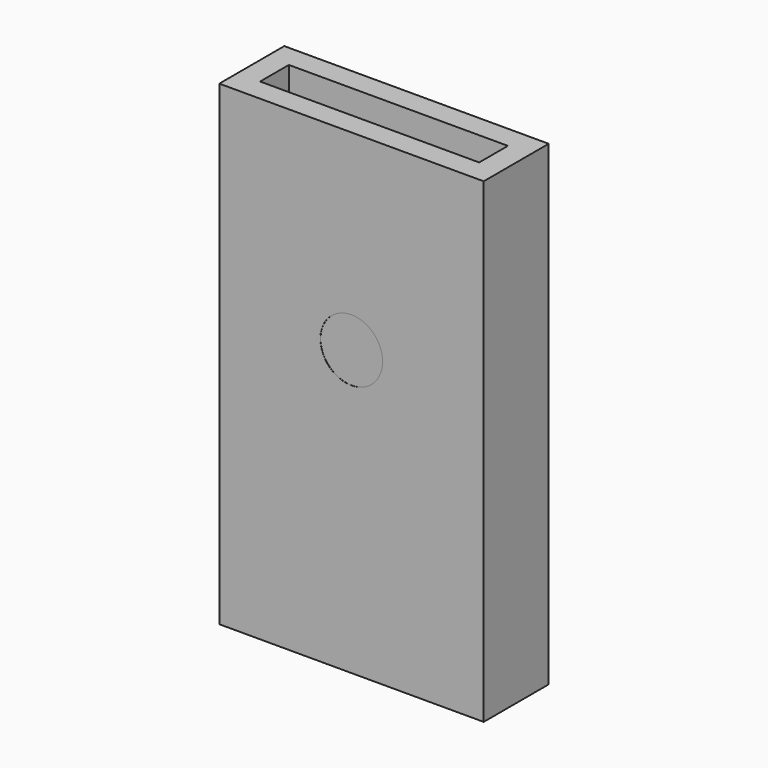
from build123d import *

# Parameters (mm, degrees)
F0_W     = 127
F0_H     = 39.0351824462
F1_DEPTH = 228.6
F2_T     = -10.8857142857
F3_R     = 14.9416499322
F4_DEPTH = 0.0762


# Not quite as in the source:
# - a length typed as a fraction of an inch, garbled in the dataset ("3 / 203.2 mm" for 3/8 in), is restored


with BuildPart() as f1:
    # F0 (on Top) → F1 (new body)
    with BuildSketch(Plane.XY):
        Rectangle(F0_W, F0_H)
    extrude(amount=F1_DEPTH)

    # F2
    f2_openings = [f1.faces().sort_by_distance(p)[0] for p in [
        (0, 0, 228.6),
    ]]
    offset(amount=F2_T, openings=f2_openings)

    # F3 (on face) → F4 (cut)
    with BuildSketch(Plane.XZ.offset(19.5175912231)):
        with Locations((0, 136.5711838007)):
            Circle(F3_R)
    extrude(amount=-F4_DEPTH, mode=Mode.SUBTRACT)


solid = f1.part
